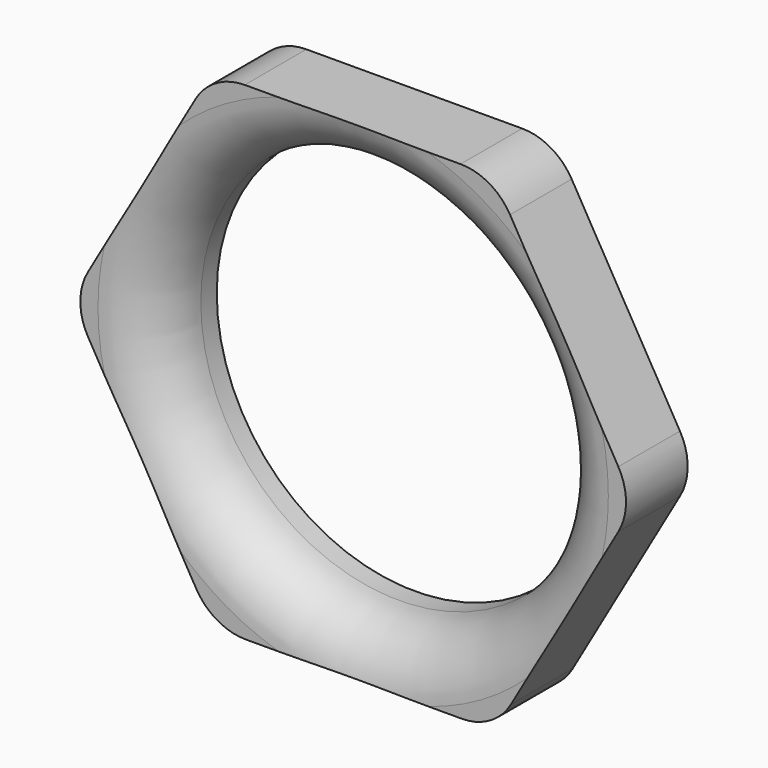
from build123d import *

# Parameters (mm, degrees)
F0_R        = 17.6278331086
F1_DEPTH    = 6.858
F2_T1_DEPTH = 21.5226968374


# Not quite as in the source:
# - a fillet or chamfer that OpenCascade refuses, or shapes differently, is made with other operations: its cross-section is extruded or revolved along the edge and cut away or added


with BuildPart() as f1:
    # F0 (on Front) → F1 (new body)
    with BuildSketch(Plane.XZ):
        Polygon((25.0675420445, 0.0543576147), (12.486695947, 21.7363070283), (-12.5808460975, 21.6819494136), (-25.0675420445, -0.0543576147), (-12.486695947, -21.7363070283), (12.5808460975, -21.6819494136), align=None)
        Circle(F0_R, mode=Mode.SUBTRACT)
    extrude(amount=F1_DEPTH)

    # F2: fillet of radius 5.08 on 7 edges, made by hand

    # F2_s2 → F2_t1 (cut)
    with BuildSketch(Plane.XZ.offset(-7.3323484187)):
        with BuildLine():
            ThreePointArc((-23.6065836488, 2.4888163666), (-24.2816651572, -0.052653483), (-23.5955679683, -2.5911716899))
            Line((-23.5955679683, -2.5911716899), (-25.0675420445, -0.0543576147))
            Line((-25.0675420445, -0.0543576147), (-23.6065836488, 2.4888163666))
        make_face()
        with BuildLine():
            ThreePointArc((-13.9586700232, -19.1994929531), (-12.0952333247, -21.0548656138), (-9.5537634751, -21.7299471223))
            Line((-9.5537634751, -21.7299471223), (-12.486695947, -21.7363070283))
            Line((-12.486695947, -21.7363070283), (-13.9586700232, -19.1994929531))
        make_face()
        with BuildLine():
            ThreePointArc((14.0418044932, -19.1387754323), (12.1864318325, -21.0022121308), (9.6479136256, -21.6883093197))
            Line((9.6479136256, -21.6883093197), (12.5808460975, -21.6819494136))
            Line((12.5808460975, -21.6819494136), (14.0418044932, -19.1387754323))
        make_face()
        with BuildLine():
            ThreePointArc((23.6065836488, -2.4888163666), (24.2816651572, 0.052653483), (23.5955679683, 2.5911716899))
            Line((23.5955679683, 2.5911716899), (25.0675420445, 0.0543576147))
            Line((25.0675420445, 0.0543576147), (23.6065836488, -2.4888163666))
        make_face()
        with BuildLine():
            ThreePointArc((13.9586700232, 19.1994929531), (12.0952333247, 21.0548656138), (9.5537634751, 21.7299471223))
            Line((9.5537634751, 21.7299471223), (12.486695947, 21.7363070283))
            Line((12.486695947, 21.7363070283), (13.9586700232, 19.1994929531))
        make_face()
        with BuildLine():
            ThreePointArc((-9.6479136256, 21.6883093197), (-12.1864318325, 21.0022121308), (-14.0418044932, 19.1387754323))
            Line((-14.0418044932, 19.1387754323), (-12.5808460975, 21.6819494136))
            Line((-12.5808460975, 21.6819494136), (-9.6479136256, 21.6883093197))
        make_face()
    extrude(amount=F2_T1_DEPTH, mode=Mode.SUBTRACT)

    # F2_s3 → F2_t4 (revolve, cut)
    with BuildSketch(Plane.XY):
        with BuildLine():
            ThreePointArc((17.6278331086, -1.778), (19.1157306602, -5.3701024484), (22.7078331086, -6.858))
            Line((22.7078331086, -6.858), (17.6278331086, -6.858))
            Line((17.6278331086, -6.858), (17.6278331086, -1.778))
        make_face()
    revolve(axis=Axis((0, -6.858, 0), (0, -1, 0)), mode=Mode.SUBTRACT)


solid = f1.part
